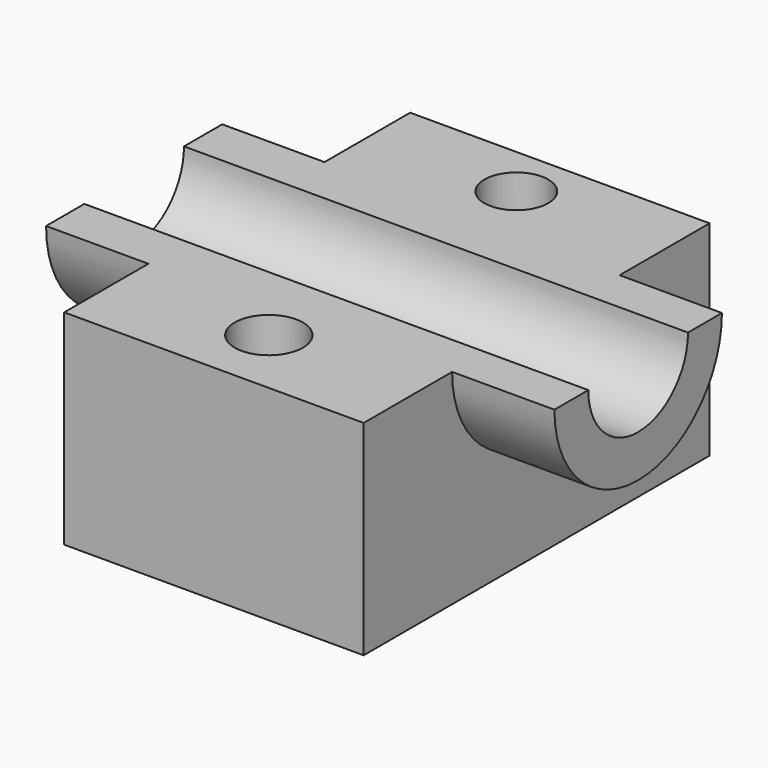
from build123d import *

# Parameters (mm, degrees)
F0_W     = 74.3527244776
F0_H     = 107.3727235198
F0_R     = 8.4778544631
F0_R_2   = 7.9454205322
F1_DEPTH = 50.8
F3_DEPTH = 25.4
F4_DEPTH = 76.2
F6_DEPTH = 25.4


with BuildPart() as f1:
    # F0 (on Top) → F1 (new body)
    with BuildSketch(Plane.XY):
        with Locations((-6.234546192, 0.2309083939)):
            Rectangle(F0_W, F0_H)
        with Locations((-6.4654541202, -36.1372716725)):
            Circle(F0_R, mode=Mode.SUBTRACT)
        with Locations((-6.6963643767, 40.9863628447)):
            Circle(F0_R_2, mode=Mode.SUBTRACT)
    extrude(amount=F1_DEPTH)

    # F2 (on face) → F3 (join)
    with BuildSketch(Plane(origin=(-43.4109084308, 0, 0), x_dir=(0, -1, 0), z_dir=(-1, 0, 0))):
        with BuildLine():
            ThreePointArc((-27.3364075131, 50.8), (0, 23.4635924869), (27.3364075131, 50.8))
            Line((27.3364075131, 50.8), (15.4696153843, 50.8))
            ThreePointArc((15.4696153843, 50.8), (0, 35.3303846157), (-15.4696153843, 50.8))
            Line((-15.4696153843, 50.8), (-27.3364075131, 50.8))
        make_face()
    extrude(amount=F3_DEPTH)

    # F4 (cut): a face of the model
    f4_faces = [f1.faces().sort_by_distance(p)[0] for p in [
        (-43.4109084308, 0, 44.234491317),
    ]]
    extrude(f4_faces, amount=-F4_DEPTH, mode=Mode.SUBTRACT)

    # F5 (on face) → F6 (join)
    with BuildSketch(Plane.YZ.offset(30.9418160468)):
        with BuildLine():
            ThreePointArc((-25.9977905066, 50.8), (0, 24.8022094934), (25.9977905066, 50.8))
            Line((25.9977905066, 50.8), (15.4696153843, 50.8))
            ThreePointArc((15.4696153843, 50.8), (0, 35.3303846157), (-15.4696153843, 50.8))
            Line((-15.4696153843, 50.8), (-25.9977905066, 50.8))
        make_face()
    extrude(amount=F6_DEPTH)


solid = f1.part
